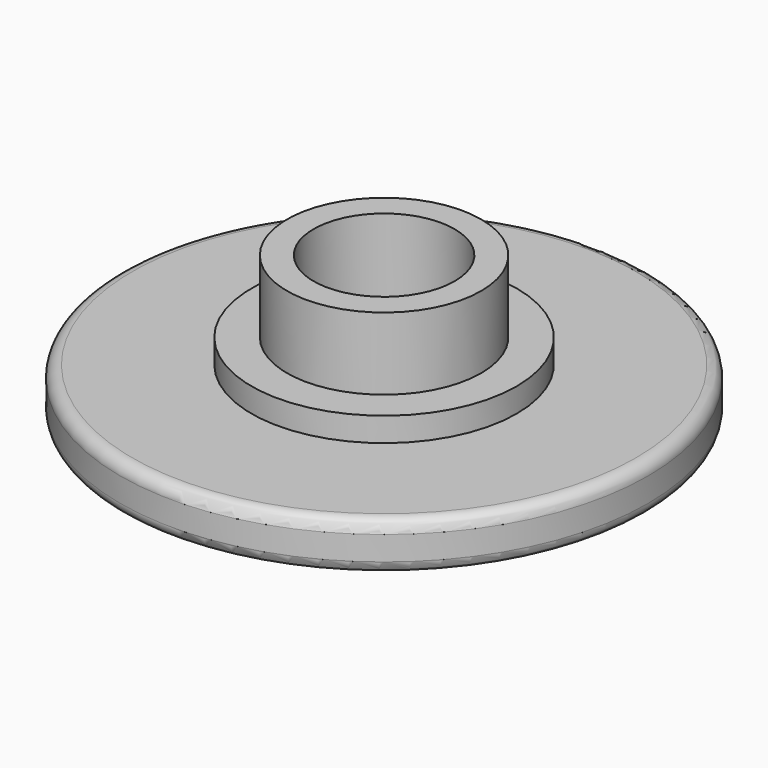
from build123d import *

# Parameters (mm, degrees)
F0_R          = 10.95
F0_R_2        = 0.069
F3_DEPTH      = 2
F1_R          = 5.5
F4_DEPTH      = 3
F2_R          = 4.025
F5_DEPTH      = 6
F6_R          = 0.5
F7_R          = 2.9249999207
F8_DEPTH      = 4
F10_TEXT_SIZE = 14.7185275435
F11_DEPTH     = 1


# Not quite as in the source:
# - Text() gives the source's letters only with a copy of the font that has no kerning and outlines rounded to 1/6400 em; it was checked with that copy


with BuildPart() as f3:
    # F0 (on Top) → F3 (new body)
    with BuildSketch(Plane.XY):
        Circle(F0_R)
        Circle(F0_R_2, mode=Mode.SUBTRACT)
    extrude(amount=F3_DEPTH)

    # F1 (on Top) → F4 (join)
    with BuildSketch(Plane.XY):
        Circle(F1_R)
    extrude(amount=F4_DEPTH)

    # F2 (on Top) → F5 (join)
    with BuildSketch(Plane.XY):
        Circle(F2_R)
    extrude(amount=F5_DEPTH)

    # F6
    f6_edges = [f3.edges().sort_by_distance(p)[0] for p in [
        (10.95, 0, 1),
        (-10.95, 0, 0),
        (-10.95, 0, 2),
    ]]
    fillet(f6_edges, radius=F6_R)

    # F7 (on face) → F8 (cut)
    with BuildSketch(Plane.XY.offset(6)):
        Circle(F7_R)
    extrude(amount=-F8_DEPTH, mode=Mode.SUBTRACT)

    # F10 (on face) → F11 (cut)
    with BuildSketch(Plane(origin=(0, 0, 0), x_dir=(1, 0, 0), z_dir=(0, 0, -1))):
        with Locations((-9.3440155615, -5.4595139809)):
            Text('EO', F10_TEXT_SIZE, font='Open Sans', text_align=(TextAlign.LEFT, TextAlign.BOTTOM))
    extrude(amount=-F11_DEPTH, mode=Mode.SUBTRACT)


solid = f3.part
